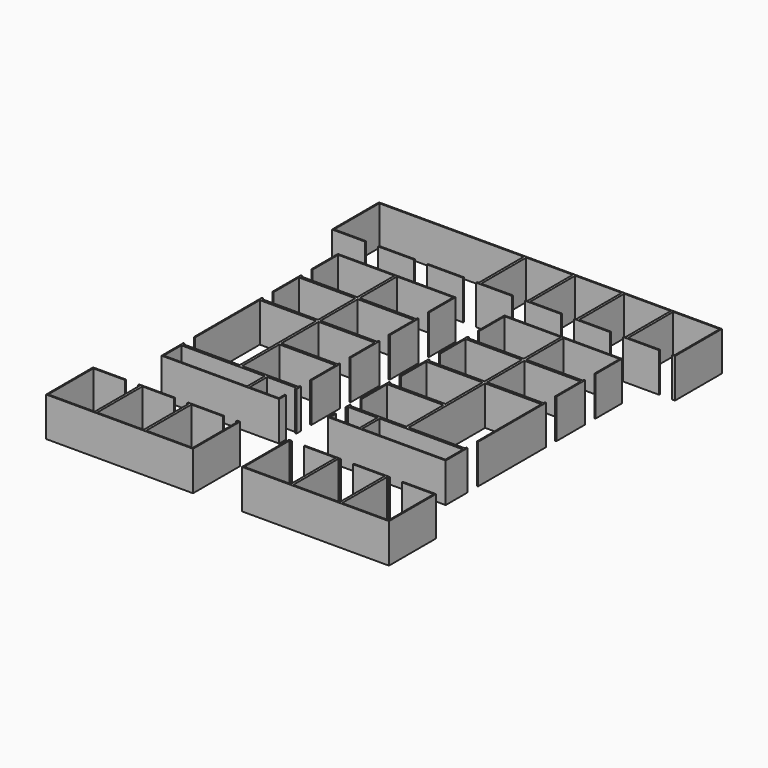
from build123d import *

# Parameters (mm, degrees)
F1_DEPTH = 2438.4
F0_W     = 5184.6479174943
F0_H     = 1371.6


# Not quite as in the source:
# - a feature names something its author has since deleted; it is built from what else it names


with BuildPart() as f1:
    # F0 (on Top) → F1 (new body)
    with BuildSketch(Plane.XY):
        Polygon((7664.9965142406, 1464.8489384322), (7664.9965142406, -2192.7510615678), (10712.9965142406, -2192.7510615678), (10712.9965142406, 1464.8489384322), (8655.5965142406, 1464.8489384322), (8655.5965142406, 1388.6489384322), (10636.7965142406, 1388.6489384322), (10636.7965142406, -2116.5510615678), (7741.1965142406, -2116.5510615678), (7741.1965142406, 1388.6489384322), (7842.7965142406, 1388.6489384322), (7842.7965142406, 1464.8489384322), align=None)
        Polygon((10712.9965142406, 1464.8489384322), (10712.9965142406, -2192.7510615678), (13760.9965142406, -2192.7510615678), (13760.9965142406, 1464.8489384322), (11703.5965142406, 1464.8489384322), (11703.5965142406, 1388.6489384322), (13684.7965142406, 1388.6489384322), (13684.7965142406, -2116.5510615678), (10789.1965142406, -2116.5510615678), (10789.1965142406, 1388.6489384322), (10890.7965142406, 1388.6489384322), (10890.7965142406, 1464.8489384322), align=None)
        Polygon((13760.9965142406, 1464.8489384322), (13760.9965142406, -2192.7510615678), (16808.9965142406, -2192.7510615678), (16808.9965142406, 1464.8489384322), (14751.5965142406, 1464.8489384322), (14751.5965142406, 1388.6489384322), (16732.7965142406, 1388.6489384322), (16732.7965142406, -2116.5510615678), (13837.1965142406, -2116.5510615678), (13837.1965142406, 1388.6489384322), (13938.7965142406, 1388.6489384322), (13938.7965142406, 1464.8489384322), align=None)
    extrude(amount=F1_DEPTH)


with BuildPart() as f1b:
    # F0 (on Top) → F1, piece 2 (new body)
    with BuildSketch(Plane.XY):
        Polygon((7664.9965142406, 6207.1020367294), (7664.9965142406, 6029.3020367294), (9643.1485967463, 6029.3020367294), (11322.5965142406, 6029.3020367294), (11322.5965142406, 9077.3020367294), (7664.9965142406, 9077.3020367294), (7664.9965142406, 7019.9020367294), (7741.1965142406, 7019.9020367294), (7741.1965142406, 9001.1020367294), (11246.3965142407, 9001.1020367294), (11246.3965142406, 6105.5020367294), (7741.1965142406, 6105.5020367294), (7741.1965142406, 6207.1020367294), align=None)
        Polygon((9643.1485967463, 6029.3020367294), (7664.9965142406, 6029.3020367294), (7664.9965142406, 5851.5020367294), (7741.1965142406, 5851.5020367294), (7741.1965142406, 5953.1020367294), (9566.9485967463, 5953.1020367294), (9566.9485967463, 4581.5020367294), (7741.1965142406, 4581.5020367294), (7741.1965142406, 5038.7020367294), (7664.9965142406, 5038.7020367294), (7664.9965142406, 4505.3020367294), (9643.1485967463, 4505.3020367294), align=None)
        Polygon((11322.5965142406, 6029.3020367294), (9643.1485967463, 6029.3020367294), (9643.1485967463, 4505.3020367294), (13002.0444317349, 4505.3020367294), (14980.1965142406, 4505.3020367294), (14980.1965142406, 6029.3020367294), (13002.0444317349, 6029.3020367294), align=None)
        with Locations((12311.6725554935, 5267.3020367294)):
            Rectangle(F0_W, F0_H, mode=Mode.SUBTRACT)
        Polygon((11322.5965142406, 9077.3020367294), (11322.5965142406, 6029.3020367294), (13002.0444317349, 6029.3020367294), (14980.1965142406, 6029.3020367294), (14980.1965142406, 6207.1020367294), (14903.9965142406, 6207.1020367294), (14903.9965142406, 6105.5020367294), (11398.7965142406, 6105.5020367294), (11398.7965142406, 9077.3020367294), (11398.7965142406, 12049.1027832031), (14903.9965142406, 12049.1027832031), (14903.9965142406, 7019.9020367294), (14980.1965142406, 7019.9020367294), (14980.1965142406, 12125.3027832031), (11322.5965142406, 12125.3027832031), (11322.5965142406, 12125.3020367294), align=None)
        Polygon((7664.9965142406, 9077.3020367294), (11322.5965142406, 9077.3020367294), (11322.5965142406, 12125.3020367294), (11322.5965142406, 12125.3027832031), (7664.9965142406, 12125.3027832031), (7664.9965142406, 10067.9020367294), (7741.1965142406, 10067.9020367294), (7741.1965142406, 12049.1020367294), (11246.3965142406, 12049.1020367294), (11246.3965142406, 9153.5020367294), (7741.1965142406, 9153.5020367294), (7741.1965142406, 9255.1020367294), (7664.9965142406, 9255.1020367294), align=None)
        Polygon((7664.9965142406, 12125.3027832031), (11322.5965142406, 12125.3027832031), (11322.5965142406, 14975.1817123413), (11322.5965142406, 15173.3020367294), (7664.9965142406, 15173.3020367294), (7664.9965142406, 14975.1817123413), (7664.9965142406, 13115.9020367294), (7741.1965142406, 13115.9020367294), (7741.1965142406, 15097.1020367294), (11246.3965142406, 15097.1020367294), (11246.3965142406, 12201.5020367294), (7741.1965142406, 12201.5020367294), (7741.1965142406, 12303.1020367294), (7664.9965142406, 12303.1020367294), align=None)
        Polygon((11322.5965142406, 14975.1817123413), (11322.5965142406, 12125.3027832031), (14980.1965142406, 12125.3027832031), (14980.1965142406, 12303.1020367294), (14903.9965142406, 12303.1020367294), (14903.9965142406, 12201.5020367294), (11398.7965142406, 12201.5020367294), (11398.7965142406, 15097.1020367294), (14903.9965142406, 15097.1020367294), (14903.9965142406, 13115.9020367294), (14980.1965142406, 13115.9020367294), (14980.1965142406, 14975.1817123413), (14980.1965142406, 15173.3020367294), (11322.5965142406, 15173.3020367294), align=None)
        Polygon((7664.9965142406, 15173.3020367294), (11322.5965142406, 15173.3020367294), (11322.5965142406, 18221.3020367294), (7664.9965142406, 18221.3020367294), (7664.9965142406, 16163.9020367294), (7741.1965142406, 16163.9020367294), (7741.1965142406, 18145.1020367294), (11246.3965142406, 18145.1020367294), (11246.3965142406, 15249.5020367294), (7741.1965142406, 15249.5020367294), (7741.1965142406, 15351.1020367294), (7664.9965142406, 15351.1020367294), align=None)
        Polygon((11322.5965142406, 18221.3020367294), (11322.5965142406, 15173.3020367294), (14980.1965142406, 15173.3020367294), (14980.1965142406, 15351.1020367294), (14903.9965142406, 15351.1020367294), (14903.9965142406, 15249.5020367294), (11398.7965142406, 15249.5020367294), (11398.7965142406, 18145.1020367294), (14903.9965142406, 18145.1020367294), (14903.9965142406, 16163.9020367294), (14980.1965142406, 16163.9020367294), (14980.1965142406, 18221.3020367294), align=None)
    extrude(amount=F1_DEPTH)


with BuildPart() as f1c:
    # F0 (on Top) → F1, piece 3 (new body)
    with BuildSketch(Plane.XY):
        Polygon((7665.0528568344, 23707.5518684133), (7665.0504387024, 23707.5518684133), (7665.0504387024, 20049.9518684133), (9722.4504387024, 20049.9518684133), (9722.4504387024, 20126.1518684133), (7741.2504387024, 20126.1518684133), (7741.2504387024, 23631.3518684133), (10636.8504387024, 23631.3518684133), (10636.8504387024, 20126.1518684133), (10535.2504387024, 20126.1518684133), (10535.2504387024, 20049.9518684133), (10713.0504387024, 20049.9518684133), (10713.0504387024, 23707.5518684133), align=None)
        Polygon((7665.0504387024, 20049.9518684133), (7665.0504387024, 23707.5518684133), (4617.0528568344, 23707.5518684133), (4617.0504387024, 23707.5518684133), (4617.0504387024, 20049.9518684133), (6674.4504387024, 20049.9518684133), (6674.4504387024, 20126.1518684133), (4693.2504387024, 20126.1518684133), (4693.2504387024, 23631.3518684133), (7588.8504387024, 23631.3518684133), (7588.8504387024, 20126.1518684133), (7487.2504387024, 20126.1518684133), (7487.2504387024, 20049.9518684133), align=None)
        Polygon((4617.0504387024, 20049.9518684133), (4617.0504387024, 23707.5518684133), (1569.0504387024, 23707.5518684133), (-1478.9495612976, 23707.5518684133), (-4526.9495612976, 23707.5518684133), (-4526.9495612976, 20049.9518684133), (-2469.5495612976, 20049.9518684133), (-2469.5495612976, 20126.1518684133), (-4450.7495612976, 20126.1518684133), (-4450.7495612976, 23631.3518684133), (-1555.1495612976, 23631.3518684133), (-1402.7495612976, 23631.3518684133), (1492.8504387024, 23631.3518684133), (1645.2504387024, 23631.3518684133), (4540.8504387024, 23631.3518684133), (4540.8504387024, 20126.1518684133), (4439.2504387024, 20126.1518684133), (4439.2504387024, 20049.9518684133), align=None)
        Polygon((10713.0528568344, 23707.5518684133), (10713.0504387024, 23707.5518684133), (10713.0504387024, 20049.9518684133), (12770.4504387024, 20049.9518684133), (12770.4504387024, 20126.1518684133), (10789.2504387024, 20126.1518684133), (10789.2504387024, 23631.3518684133), (13684.8504387024, 23631.3518684133), (13684.8504387024, 20126.1518684133), (13583.2504387024, 20126.1518684133), (13583.2504387024, 20049.9518684133), (13761.0504387024, 20049.9518684133), (13761.0504387024, 23707.5518684133), align=None)
        Polygon((13761.0528568344, 23707.5518684133), (13761.0504387024, 23707.5518684133), (13761.0504387024, 20049.9518684133), (15818.4504387024, 20049.9518684133), (15818.4504387024, 20126.1518684133), (13837.2504387024, 20126.1518684133), (13837.2504387024, 23631.3518684133), (16732.8504387024, 23631.3518684133), (16732.8504387024, 20126.1518684133), (16631.2504387024, 20126.1518684133), (16631.2504387024, 20049.9518684133), (16809.0504387024, 20049.9518684133), (16809.0504387024, 23707.5518684133), align=None)
    extrude(amount=F1_DEPTH)


with BuildPart() as f1d:
    # F0 (on Top) → F1, piece 4 (new body)
    with BuildSketch(Plane.XY):
        Polygon((1569.0504387024, 20049.9518684133), (3626.4504387024, 20049.9518684133), (3626.4504387024, 20126.1518684133), (1645.2504387024, 20126.1518684133), (1492.8504387024, 20126.1518684133), (1391.2504387024, 20126.1518684133), (1391.2504387024, 20049.9518684133), align=None)
    extrude(amount=F1_DEPTH)


with BuildPart() as f1e:
    # F0 (on Top) → F1, piece 5 (new body)
    with BuildSketch(Plane.XY):
        Polygon((-1478.9495612976, 20049.9518684133), (578.4504387024, 20049.9518684133), (578.4504387024, 20126.1518684133), (-1402.7495612976, 20126.1518684133), (-1555.1495612976, 20126.1518684133), (-1656.7495612976, 20126.1518684133), (-1656.7495612976, 20049.9518684133), align=None)
    extrude(amount=F1_DEPTH)


with BuildPart() as f1f:
    # F0 (on Top) → F1, piece 6 (new body)
    with BuildSketch(Plane.XY):
        Polygon((-2622.0034857594, 6105.5020367294), (-2622.0034857594, 6207.1020367294), (-2698.2034857594, 6207.1020367294), (-2698.2034857594, 6029.3020367294), (-720.0514032537, 6029.3020367294), (959.3965142406, 6029.3020367294), (959.3965142406, 9077.3020367294), (959.3965142406, 12125.3020367294), (959.3965142406, 12125.3027832031), (-2698.2034857594, 12125.3027832031), (-2698.2034857594, 7019.9020367294), (-2622.0034857594, 7019.9020367294), (-2622.0034857594, 12049.1027832031), (883.1965142406, 12049.1027832031), (883.1965142406, 9077.3020367294), (883.1965142406, 6105.5020367294), align=None)
        Polygon((-720.0514032537, 6029.3020367294), (-2698.2034857594, 6029.3020367294), (-2698.2034857594, 4505.3020367294), (-720.0514032537, 4505.3020367294), (2638.8444317349, 4505.3020367294), (2638.8444317349, 6029.3020367294), (959.3965142406, 6029.3020367294), align=None)
        with Locations((-29.6795270123, 5267.3020367294)):
            Rectangle(F0_W, F0_H, mode=Mode.SUBTRACT)
        Polygon((-2698.2034857594, 12303.1020367294), (-2698.2034857594, 12125.3027832031), (959.3965142406, 12125.3027832031), (959.3965142406, 14975.1817123413), (959.3965142406, 15173.3020367294), (-2698.2034857594, 15173.3020367294), (-2698.2034857594, 14975.1817123413), (-2698.2034857594, 13115.9020367294), (-2622.0034857594, 13115.9020367294), (-2622.0034857594, 15097.1020367294), (883.1965142406, 15097.1020367294), (883.1965142406, 12201.5020367294), (-2622.0034857594, 12201.5020367294), (-2622.0034857594, 12303.1020367294), align=None)
        Polygon((4616.9965142406, 12125.3027832031), (959.3965142406, 12125.3027832031), (959.3965142406, 12125.3020367294), (959.3965142406, 9077.3020367294), (4616.9965142406, 9077.3020367294), (4616.9965142406, 9255.1020367294), (4540.7965142406, 9255.1020367294), (4540.7965142406, 9153.5020367294), (1035.5965142406, 9153.5020367294), (1035.5965142406, 12049.1020367294), (4540.7965142406, 12049.1020367294), (4540.7965142406, 10067.9020367294), (4616.9965142406, 10067.9020367294), align=None)
        Polygon((959.3965142406, 14975.1817123413), (959.3965142406, 12125.3027832031), (4616.9965142406, 12125.3027832031), (4616.9965142406, 12303.1020367294), (4540.7965142406, 12303.1020367294), (4540.7965142406, 12201.5020367294), (1035.5965142406, 12201.5020367294), (1035.5965142406, 15097.1020367294), (4540.7965142406, 15097.1020367294), (4540.7965142406, 13115.9020367294), (4616.9965142406, 13115.9020367294), (4616.9965142406, 14975.1817123413), (4616.9965142406, 15173.3020367294), (959.3965142406, 15173.3020367294), align=None)
        Polygon((959.3965142406, 9077.3020367294), (959.3965142406, 6029.3020367294), (2638.8444317349, 6029.3020367294), (4616.9965142406, 6029.3020367294), (4616.9965142406, 6207.1020367294), (4540.7965142406, 6207.1020367294), (4540.7965142406, 6105.5020367294), (1035.5965142406, 6105.5020367294), (1035.5965142405, 9001.1020367294), (4540.7965142406, 9001.1020367294), (4540.7965142406, 7019.9020367294), (4616.9965142406, 7019.9020367294), (4616.9965142406, 9077.3020367294), align=None)
        Polygon((4616.9965142406, 6029.3020367294), (2638.8444317349, 6029.3020367294), (2638.8444317349, 4505.3020367294), (4616.9965142406, 4505.3020367294), (4616.9965142406, 5038.7020367294), (4540.7965142406, 5038.7020367294), (4540.7965142406, 4581.5020367294), (2715.0444317349, 4581.5020367294), (2715.0444317349, 5953.1020367294), (4540.7965142406, 5953.1020367294), (4540.7965142406, 5851.5020367294), (4616.9965142406, 5851.5020367294), align=None)
        Polygon((-2698.2034857594, 15173.3020367294), (959.3965142406, 15173.3020367294), (959.3965142406, 18221.3020367294), (-2698.2034857594, 18221.3020367294), (-2698.2034857594, 16163.9020367294), (-2622.0034857594, 16163.9020367294), (-2622.0034857594, 18145.1020367294), (883.1965142406, 18145.1020367294), (883.1965142406, 15249.5020367294), (-2622.0034857594, 15249.5020367294), (-2622.0034857594, 15351.1020367294), (-2698.2034857594, 15351.1020367294), align=None)
        Polygon((959.3965142406, 18221.3020367294), (959.3965142406, 15173.3020367294), (4616.9965142406, 15173.3020367294), (4616.9965142406, 15351.1020367294), (4540.7965142406, 15351.1020367294), (4540.7965142406, 15249.5020367294), (1035.5965142406, 15249.5020367294), (1035.5965142406, 18145.1020367294), (4540.7965142406, 18145.1020367294), (4540.7965142406, 16163.9020367294), (4616.9965142406, 16163.9020367294), (4616.9965142406, 18221.3020367294), align=None)
    extrude(amount=F1_DEPTH)


with BuildPart() as f1g:
    # F0 (on Top) → F1, piece 7 (new body)
    with BuildSketch(Plane.XY):
        Polygon((1391.1965142406, 1464.8489384322), (1391.1965142406, 1388.6489384322), (1492.7965142406, 1388.6489384322), (1492.7965142406, -2116.5510615678), (-1402.8034857594, -2116.5510615678), (-1402.8034857594, 1388.6489384322), (578.3965142406, 1388.6489384322), (578.3965142406, 1464.8489384322), (-1479.0034857594, 1464.8489384322), (-1479.0034857594, -2192.7510615678), (1568.9965142406, -2192.7510615678), (1568.9965142406, 1464.8489384322), align=None)
        Polygon((3626.3965142406, 1464.8489384322), (1568.9965142406, 1464.8489384322), (1568.9965142406, -2192.7510615678), (4616.9965142406, -2192.7510615678), (4616.9965142406, 1464.8489384322), (4439.1965142406, 1464.8489384322), (4439.1965142406, 1388.6489384322), (4540.7965142406, 1388.6489384322), (4540.7965142406, -2116.5510615678), (1645.1965142406, -2116.5510615678), (1645.1965142406, 1388.6489384322), (3626.3965142406, 1388.6489384322), align=None)
        Polygon((-1479.0034857594, -2192.7510615678), (-1479.0034857594, 1464.8489384322), (-1656.8034857594, 1464.8489384322), (-1656.8034857594, 1388.6489384322), (-1555.2034857594, 1388.6489384322), (-1555.2034857594, -2116.5510615678), (-4450.8034857594, -2116.5510615678), (-4450.8034857594, 1388.6489384322), (-2469.6034857594, 1388.6489384322), (-2469.6034857594, 1464.8489384322), (-4527.0034857594, 1464.8489384322), (-4527.0034857594, -2192.7510615678), align=None)
    extrude(amount=F1_DEPTH)


solid = Compound([f1.part, f1b.part, f1c.part, f1d.part, f1e.part, f1f.part, f1g.part])
